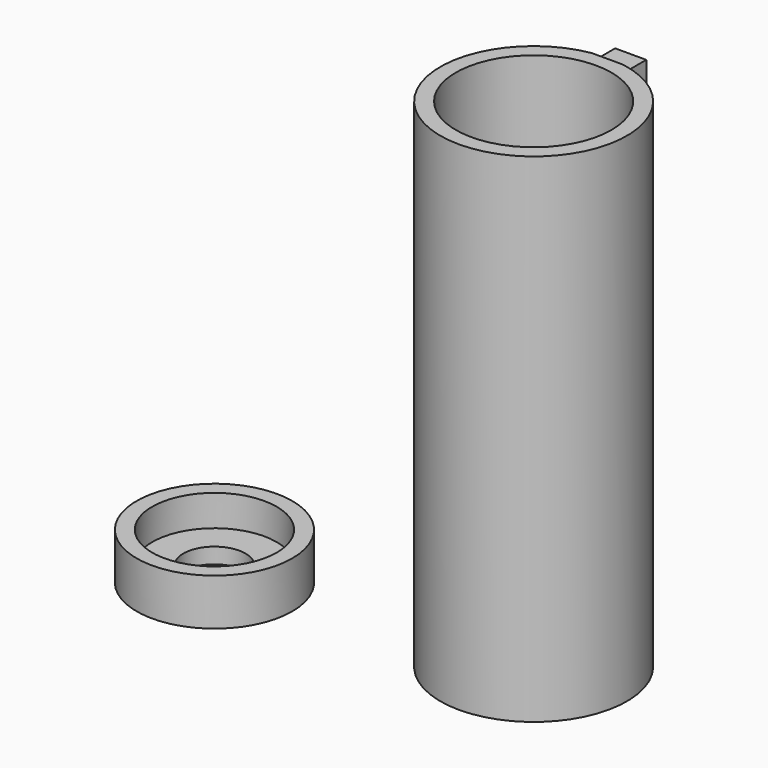
from build123d import *

# Parameters (mm, degrees)
F0_R     = 31.75
F0_R_2   = 25.4
F1_DEPTH = 19.05
F0_R_3   = 12.7
F2_DEPTH = 6.35
F3_DEPTH = 203.2
F4_W     = 12.7
F4_H     = 11.9628933773
F5_DEPTH = 3.175
F6_DEPTH = 3.175


# Not quite as in the source:
# - a feature names something its author has since deleted; it is built from what else it names


with BuildPart() as f1:
    # F0 (on Top) → F1 (new body)
    with BuildSketch(Plane.XY):
        with Locations((-115.7130011189, -18.2043969423)):
            Circle(F0_R)
        with Locations((-115.7130011189, -18.2043969423)):
            Circle(F0_R_2, mode=Mode.SUBTRACT)
    extrude(amount=F1_DEPTH)

    # F0 (on Top) → F2 (join)
    with BuildSketch(Plane.XY):
        with Locations((-115.7130011189, -18.2043969423)):
            Circle(F0_R_2)
        with Locations((-115.7130011189, -18.2043969423)):
            Circle(F0_R_3, mode=Mode.SUBTRACT)
    extrude(amount=F2_DEPTH)


with BuildPart() as f3:
    # F0 (on Top) → F3 (new body)
    with BuildSketch(Plane.XY):
        with BuildLine():
            ThreePointArc((-6.35, 37.5671066227), (-24.5934442484, -29.099355663), (38.1, 0))
            ThreePointArc((38.1, 0), (29.099355663, 24.5934442484), (6.35, 37.5671066227))
            ThreePointArc((6.35, 37.5671066227), (3.1861605167, 37.9665429182), (0, 38.1))
            ThreePointArc((0, 38.1), (-3.1861605167, 37.9665429182), (-6.35, 37.5671066227))
        make_face()
        Circle(F0_R, mode=Mode.SUBTRACT)
        with BuildLine():
            ThreePointArc((0, 38.1), (3.1861605167, 37.9665429182), (6.35, 37.5671066227))
            Line((6.35, 37.5671066227), (6.35, 49.53))
            Line((6.35, 49.53), (0, 49.53))
            Line((0, 49.53), (0, 38.1))
        make_face()
        with BuildLine():
            Line((-6.35, 49.53), (-6.35, 37.5671066227))
            ThreePointArc((-6.35, 37.5671066227), (-3.1861605167, 37.9665429182), (0, 38.1))
            Line((0, 38.1), (0, 49.53))
            Line((0, 49.53), (-6.35, 49.53))
        make_face()
    extrude(amount=F3_DEPTH)

    # F4 (on face) → F5 (cut)
    with BuildSketch(Plane.XY.offset(203.2)):
        with Locations((0, 43.5485533113)):
            Rectangle(F4_W, F4_H)
    extrude(amount=-F5_DEPTH, mode=Mode.SUBTRACT)

    # F0 (on Top) → F6 (cut)
    with BuildSketch(Plane.XY):
        with BuildLine():
            ThreePointArc((0, 38.1), (3.1861605167, 37.9665429182), (6.35, 37.5671066227))
            Line((6.35, 37.5671066227), (6.35, 49.53))
            Line((6.35, 49.53), (0, 49.53))
            Line((0, 49.53), (0, 38.1))
        make_face()
        with BuildLine():
            Line((-6.35, 49.53), (-6.35, 37.5671066227))
            ThreePointArc((-6.35, 37.5671066227), (-3.1861605167, 37.9665429182), (0, 38.1))
            Line((0, 38.1), (0, 49.53))
            Line((0, 49.53), (-6.35, 49.53))
        make_face()
    extrude(amount=F6_DEPTH, mode=Mode.SUBTRACT)


solid = Compound([f1.part, f3.part])
